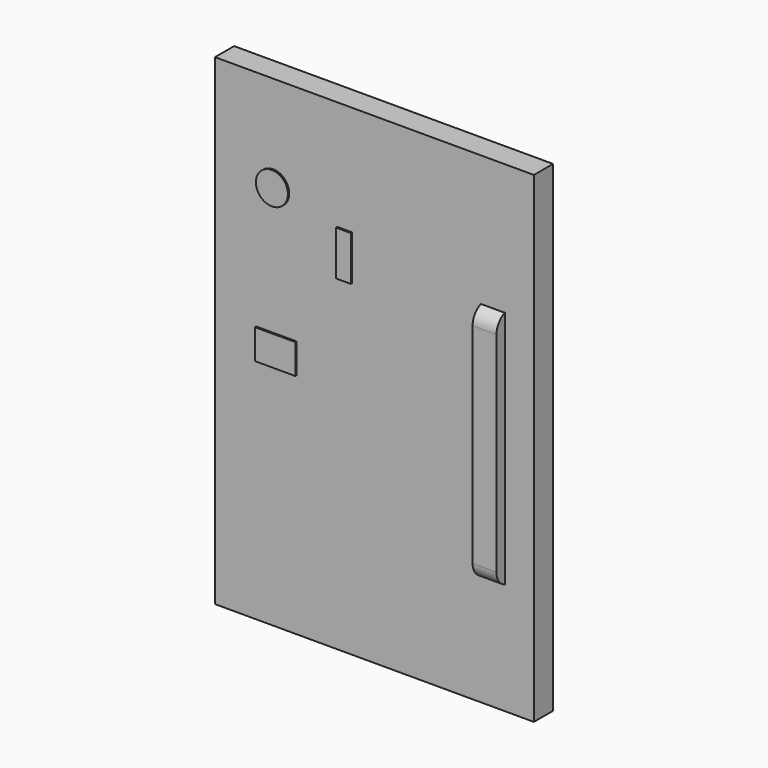
from build123d import *

# Parameters (mm, degrees)
F0_W        = 101.6
F0_H        = 7.62
F1_DEPTH    = 153.416
F2_W        = 7.62
F2_H        = 76.2
F3_DEPTH    = 3.302
F4_T1_DEPTH = 31.4134423739
F5_R        = 5.1053850436
F5_W        = 4.7544753179
F5_H        = 14.2634212971
F5_W_2      = 12.9049904644
F5_H_2      = 9.5089375973
F6_DEPTH    = 0.508


# Not quite as in the source:
# - a fillet or chamfer that OpenCascade refuses, or shapes differently, is made with other operations: its cross-section is extruded or revolved along the edge and cut away or added


with BuildPart() as f1:
    # F0 (on Top) → F1 (new body)
    with BuildSketch(Plane.XY):
        Rectangle(F0_W, F0_H)
    extrude(amount=F1_DEPTH)

    # F2 (on face) → F3 (join)
    with BuildSketch(Plane.XZ.offset(3.81)):
        with Locations((37.7244745995, 73.6427996308)):
            Rectangle(F2_W, F2_H)
    extrude(amount=F3_DEPTH)

    # F4: fillet of radius 5.08 on 2 edges, made by hand

    # F4_s2 → F4_t1 (cut)
    with BuildSketch(Plane.YZ.offset(22.0177534125)):
        with BuildLine():
            ThreePointArc((-3.81, 111.7427996308), (-6.2056458882, 109.8801567357), (-7.112, 106.984111156))
            Line((-7.112, 106.984111156), (-7.112, 111.7427996308))
            Line((-7.112, 111.7427996308), (-3.81, 111.7427996308))
        make_face()
        with BuildLine():
            ThreePointArc((-3.81, 35.5427996308), (-6.2056458882, 37.4054425258), (-7.112, 40.3014881055))
            Line((-7.112, 40.3014881055), (-7.112, 35.5427996308))
            Line((-7.112, 35.5427996308), (-3.81, 35.5427996308))
        make_face()
    extrude(amount=F4_T1_DEPTH, mode=Mode.SUBTRACT)

    # F5 (on face) → F6 (join)
    with BuildSketch(Plane.XZ.offset(3.81)):
        with Locations((-32.2624817491, 122.8942871094)):
            Circle(F5_R)
        with Locations((-9.5089431852, 111.3477125764)):
            Rectangle(F5_W, F5_H)
        with Locations((-31.2436651438, 77.3872062564)):
            Rectangle(F5_W_2, F5_H_2)
    extrude(amount=F6_DEPTH)


solid = f1.part
